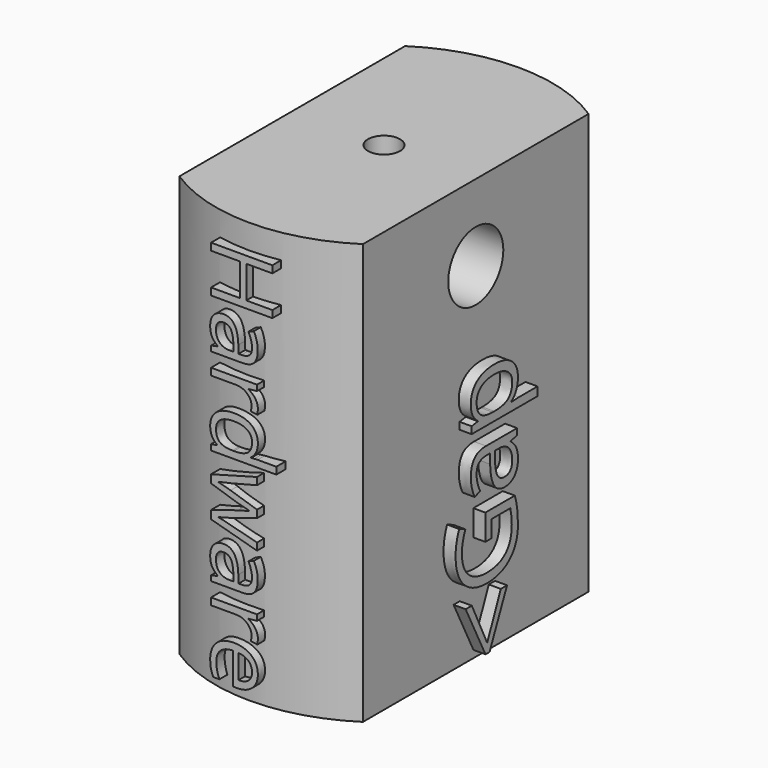
from build123d import *

# Parameters (mm, degrees)
F0_R          = 1.3335
F1_DEPTH      = 34.925
F2_R          = 2.8575
F3_DEPTH      = 7.62
F4_R          = 2.8575
F5_DEPTH      = 7.62
F6_TEXT_SIZE  = 8.8194444444
F7_DEPTH      = 1
F8_TEXT_SIZE  = 8.8194444444
F9_DEPTH      = 1
F11_TEXT_SIZE = 7.1305462766
F12_DEPTH     = 4.5


# Not quite as in the source:
# - Text() gives the source's letters only with a copy of the font that has no kerning and outlines rounded to 1/6400 em; it was checked with that copy


with BuildPart() as f1:
    # F0 (on Top) → F1 (new body)
    with BuildSketch(Plane.XY):
        with BuildLine():
            Line((-7.62, 11.7088214608), (-7.62, -11.7088214608))
            ThreePointArc((-7.62, -11.7088214608), (0, -13.97), (7.62, -11.7088214608))
            Line((7.62, -11.7088214608), (7.62, 11.7088214608))
            ThreePointArc((7.62, 11.7088214608), (0, 13.97), (-7.62, 11.7088214608))
        make_face()
        Circle(F0_R, mode=Mode.SUBTRACT)
    extrude(amount=F1_DEPTH)

    # F2 (on Right) → F3 (cut, through all)
    with BuildSketch(Plane.YZ):
        with Locations((0, 28.575)):
            Circle(F2_R)
    extrude(amount=F3_DEPTH, mode=Mode.SUBTRACT)

    # F4 (on Right) → F5 (cut, through all)
    with BuildSketch(Plane.YZ):
        with Locations((0, 6.35)):
            Circle(F4_R)
    extrude(amount=-F5_DEPTH, mode=Mode.SUBTRACT)

    # F6 (on face) → F7 (join)
    with BuildSketch(Plane(origin=(-7.62, 0, 0), x_dir=(0, -1, 0), z_dir=(-1, 0, 0))):
        with Locations(Location((3.7399669673, 30.3943946801), (0, 0, -90))):
            Text('<No', F6_TEXT_SIZE, font='Open Sans', text_align=(TextAlign.LEFT, TextAlign.BOTTOM))
        with Locations(Location((-8.2544774772, 28.1027171628), (0, 0, -90))):
            Text('Gap', F6_TEXT_SIZE, font='Open Sans', text_align=(TextAlign.LEFT, TextAlign.BOTTOM))
    extrude(amount=F7_DEPTH)

    # F8 (on face) → F9 (join)
    with BuildSketch(Plane.YZ.offset(7.62)):
        with Locations(Location((3.0399855273, 0.1541516324), (0, 0, 90))):
            Text('<Gap', F8_TEXT_SIZE, font='Open Sans', text_align=(TextAlign.LEFT, TextAlign.BOTTOM))
    extrude(amount=F9_DEPTH)

    # F11 (on offset) → F12 (join)
    with BuildSketch(Plane.XZ.offset(10.16)):
        with Locations(Location((-2.6330047637, 33.5979685334), (0, 0, -90))):
            Text('Hardware', F11_TEXT_SIZE, font='Open Sans', text_align=(TextAlign.LEFT, TextAlign.BOTTOM))
    extrude(amount=F12_DEPTH)


solid = f1.part
